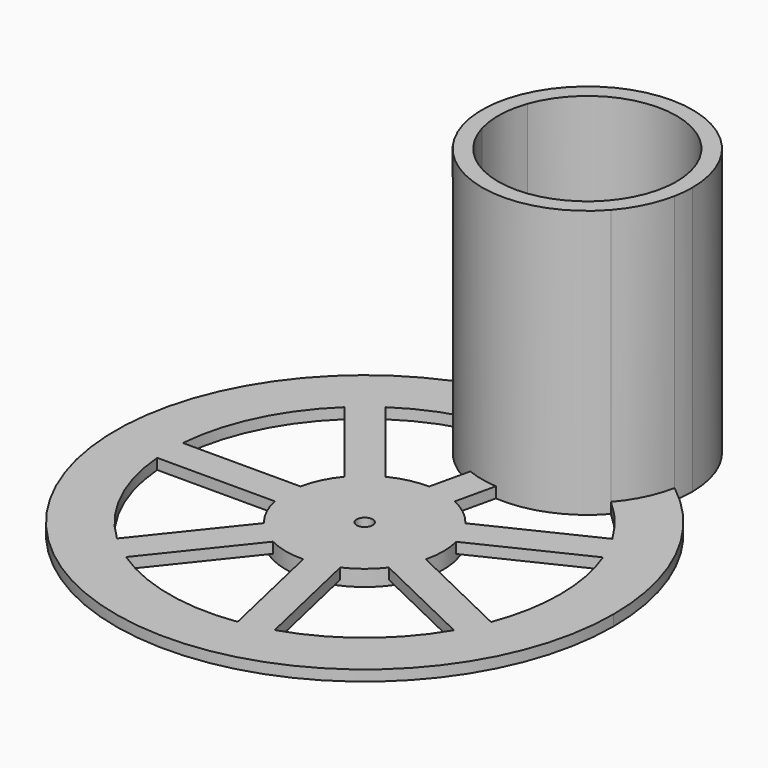
from build123d import *

# Parameters (mm, degrees)
F1_DEPTH = 2
F0_R     = 5
F0_R_2   = 1.5
F2_DEPTH = 2
F3_COUNT = 7
F4_DEPTH = 25
F5_DEPTH = 50
F6_DEPTH = 1


with BuildPart() as f1:
    # F0 (on Top) → F1 (new body)
    with BuildSketch(Plane.XY):
        with BuildLine():
            ThreePointArc((-9.6980178026, 35.1732821843), (-10.4180475342, 40.3053577212), (-9.7713618559, 45.4471900565))
            ThreePointArc((-9.7713618559, 45.4471900565), (-29.212132235, -36.1604469944), (46.4857676773, 0))
            ThreePointArc((46.4857676773, 0), (41.7541400396, 20.4332666527), (28.5224895833, 36.7068683562))
            ThreePointArc((28.5224895833, 36.7068683562), (26.8741758072, 31.793651098), (23.9987273116, 27.4822200037))
            ThreePointArc((23.9987273116, 27.4822200037), (33.217640994, 15.0930333501), (36.4857688546, 0))
            ThreePointArc((36.4857688546, 0), (1.5012714069, -36.4548695386), (-36.3622239269, -3))
            ThreePointArc((-36.3622239269, -3), (-36.4857688546, 0), (-36.3622239269, 3))
            ThreePointArc((-36.3622239269, 3), (-28.0921072309, 23.2818564603), (-9.6980178026, 35.1732821843))
        make_face()
    extrude(amount=F1_DEPTH)



with BuildPart() as f1b:
    # F0 (on Top) → F1, piece 2 (new body)
    with BuildSketch(Plane.XY):
        with BuildLine():
            ThreePointArc((14.7, 0), (1.5079551369, 14.6224509336), (-14.3906219463, 3))
            ThreePointArc((-14.3906219463, 3), (-14.7, 0), (-14.3906219463, -3))
            ThreePointArc((-14.3906219463, -3), (1.5079551369, -14.6224509336), (14.7, 0))
        make_face()
        Circle(F0_R, mode=Mode.SUBTRACT)
        Circle(F0_R)
        Circle(F0_R_2, mode=Mode.SUBTRACT)
    extrude(amount=F1_DEPTH)


with BuildPart() as f2:
    # F0 (on Top) → F2 (new body)
    with BuildSketch(Plane.XY):
        with BuildLine():
            Line((-14.3906219463, 3), (-36.3622239269, 3))
            ThreePointArc((-36.3622239269, 3), (-36.4857688546, 0), (-36.3622239269, -3))
            Line((-36.3622239269, -3), (-14.3906219463, -3))
            ThreePointArc((-14.3906219463, -3), (-14.7, 0), (-14.3906219463, 3))
        make_face()
    extrude(amount=F2_DEPTH)


with BuildPart() as f1_1:
    add(f1.part)

    add(f1b.part)  # F3 merges F1b
    # F3: F2 ×7 about axis
    f3_axis = Axis((0, 0, 2), (0, 0, -1))
    for i in range(1, F3_COUNT):
        add(f2.part.rotate(f3_axis, i * 360 / F3_COUNT))

    # F0 (on Top) → F4 (cut)
    with BuildSketch(Plane.XY):
        with BuildLine():
            ThreePointArc((21.6570841341, 29.3629364288), (8.1188473616, 35.5709944538), (-6.7722579251, 35.851748235))
            ThreePointArc((-6.7722579251, 35.851748235), (5.5264782191, 24.2130831291), (21.6570841341, 29.3629364288))
        make_face()
    extrude(amount=F4_DEPTH, mode=Mode.SUBTRACT)

    # F0 (on Top) → F5 (join)
    with BuildSketch(Plane.XY):
        with BuildLine():
            ThreePointArc((-6.4520489204, 46.03583019), (12.0680177843, 56.8522288954), (25.8814517695, 40.4456328669))
            ThreePointArc((25.8814517695, 40.4456328669), (25.8578955004, 39.5602691783), (25.7872933477, 38.6774106986))
            ThreePointArc((25.7872933477, 38.6774106986), (27.1727600693, 37.7169419064), (28.5224895833, 36.7068683562))
            ThreePointArc((28.5224895833, 36.7068683562), (28.7915053614, 38.5676543049), (28.8814517695, 40.4456328669))
            ThreePointArc((28.8814517695, 40.4456328669), (11.7530794444, 59.9331646211), (-9.7713618559, 45.4471900565))
            ThreePointArc((-9.7713618559, 45.4471900565), (-8.117043095, 45.7716091911), (-6.4520489204, 46.03583019))
        make_face()
        with BuildLine():
            ThreePointArc((-6.7722579251, 35.851748235), (-7.4103241816, 40.9688853837), (-6.4520489204, 46.03583019))
            ThreePointArc((-6.4520489204, 46.03583019), (-8.117043095, 45.7716091911), (-9.7713618559, 45.4471900565))
            ThreePointArc((-9.7713618559, 45.4471900565), (-10.4180475342, 40.3053577212), (-9.6980178026, 35.1732821843))
            ThreePointArc((-9.6980178026, 35.1732821843), (-8.2421219769, 35.5426329108), (-6.7722579251, 35.851748235))
        make_face()
        with BuildLine():
            ThreePointArc((28.5224895833, 36.7068683562), (27.1727600693, 37.7169419064), (25.7872933477, 38.6774106986))
            ThreePointArc((25.7872933477, 38.6774106986), (24.4522045664, 33.6964711194), (21.6570841341, 29.3629364288))
            ThreePointArc((21.6570841341, 29.3629364288), (22.8472657721, 28.4466830343), (23.9987273116, 27.4822200037))
            ThreePointArc((23.9987273116, 27.4822200037), (26.8741758072, 31.793651098), (28.5224895833, 36.7068683562))
        make_face()
        with BuildLine():
            ThreePointArc((21.6570841341, 29.3629364288), (5.5264782191, 24.2130831291), (-6.7722579251, 35.851748235))
            ThreePointArc((-6.7722579251, 35.851748235), (-8.2421219769, 35.5426329108), (-9.6980178026, 35.1732821843))
            ThreePointArc((-9.6980178026, 35.1732821843), (4.8589154172, 21.2882993925), (23.9987273116, 27.4822200037))
            ThreePointArc((23.9987273116, 27.4822200037), (22.8472657721, 28.4466830343), (21.6570841341, 29.3629364288))
        make_face()
    extrude(amount=F5_DEPTH)


    add(f2.part)  # F6 merges F2
    # F0 (on Top) → F6 (join)
    with BuildSketch(Plane.XY):
        with BuildLine():
            ThreePointArc((14.7, 0), (1.5079551369, 14.6224509336), (-14.3906219463, 3))
            ThreePointArc((-14.3906219463, 3), (-14.7, 0), (-14.3906219463, -3))
            ThreePointArc((-14.3906219463, -3), (1.5079551369, -14.6224509336), (14.7, 0))
        make_face()
        Circle(F0_R, mode=Mode.SUBTRACT)
    extrude(amount=-F6_DEPTH)


solid = f1_1.part
